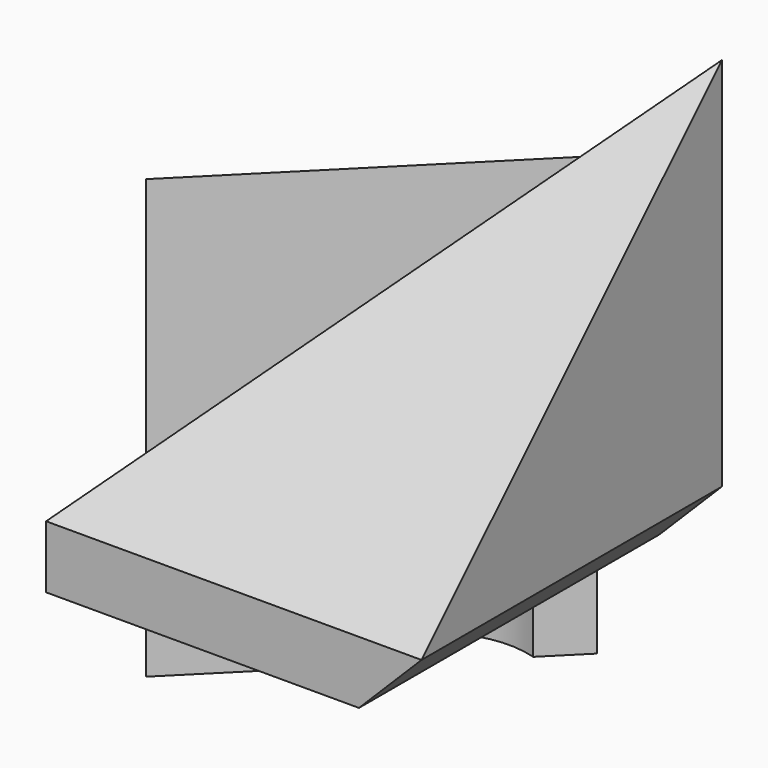
from build123d import *

# Parameters (mm, degrees)
F0_W      = 60
F0_H      = 10
F1_DEPTH  = 60
F2_SIZE   = 9.99999
F9_DEPTH  = 40
F11_DEPTH = 20
F13_R     = 15
F14_DEPTH = 26
F15_R     = 2


# Not quite as in the source:
# - a fillet or chamfer is up to 0.001 mm smaller than in the source, because OpenCascade refuses the exact size


with BuildPart() as f1:
    # F0 (on Front) → F1 (new body)
    with BuildSketch(Plane.XZ):
        with Locations((30, 5)):
            Rectangle(F0_W, F0_H)
    extrude(amount=-F1_DEPTH)

    # F2 (size 10 in the source; OpenCascade refuses exactly that, so slightly less here)
    f2_edges = [f1.edges().sort_by_distance(p)[0] for p in [
        (60, 30, 0),
    ]]
    chamfer(f2_edges, length=F2_SIZE)

    # F5 (on face) → F6 section 0
    with BuildSketch(Plane.XY.offset(10), mode=Mode.PRIVATE) as f6_s0:
        Polygon((60, 0), (60, 60), (0, 0), align=None)
    loft([f6_s0.sketch, Vertex(60, 60, 70)])

    # F8 (on face) → F9 (join)
    with BuildSketch(Plane.XY.offset(10)):
        Polygon((40, 60), (0, 60), (0, 20), align=None)
    extrude(amount=F9_DEPTH)

    # F10 (on face) → F11 (join)
    with BuildSketch(Plane(origin=(0, 0, 0), x_dir=(1, 0, 0), z_dir=(0, 0, -1))):
        Polygon((0, -20), (0, -60), (40, -60), align=None)
    extrude(amount=F11_DEPTH)

    # F9_face (on face) → F12 section 0
    with BuildSketch(Plane(origin=(13.3333333333, 46.6666666667, 50), x_dir=(1, 0, 0), z_dir=(0, 0, 1)), mode=Mode.PRIVATE) as f12_s0:
        Polygon((26.6666666667, 13.3333333333), (-13.3333333333, 13.3333333333), (-13.3333333333, -26.6666666667), align=None)
    loft([f12_s0.sketch, Vertex(0, 60, -20)], mode=Mode.SUBTRACT)

    # F13 (on face) → F14 (cut)
    with BuildSketch(Plane(origin=(0, 0, -20), x_dir=(1, 0, 0), z_dir=(0, 0, -1))):
        with Locations((30, -40)):
            Circle(F13_R)
    extrude(amount=-F14_DEPTH, mode=Mode.SUBTRACT)

    # F15
    f15_edges = [f1.edges().sort_by_distance(p)[0] for p in [
        (15, 40, 6),
    ]]
    fillet(f15_edges, radius=F15_R)


solid = f1.part
